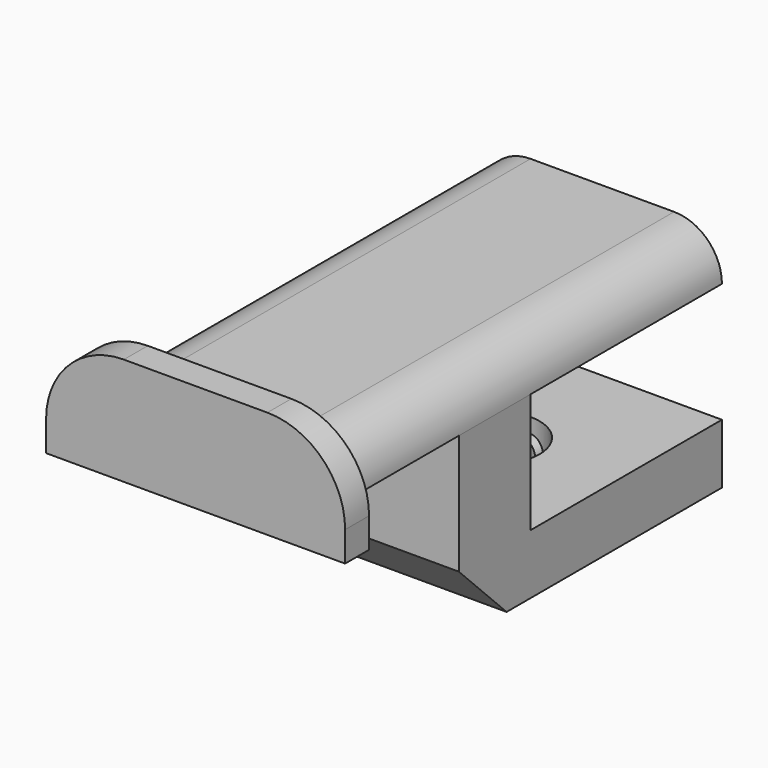
from build123d import *

# Parameters (mm, degrees)
F0_W      = 40
F0_H      = 80
F1_DEPTH  = 8
F2_W      = 40
F2_H      = 15
F3_DEPTH  = 30
F4_W      = 40
F4_H      = 10
F5_DEPTH  = 40
F6_R      = 7.99999
F7_SIZE2  = 10
F7_SIZE   = 10
F9_DEPTH  = 5
F10_W     = 48
F10_H     = 5
F10_W_2   = 1
F11_DEPTH = 5
F12_R     = 7.5
F12_R_2   = 6
F13_DEPTH = 11
F14_R     = 2.5
F15_DEPTH = 32
F16_DEPTH = 25


# Not quite as in the source:
# - a fillet or chamfer is up to 0.001 mm smaller than in the source, because OpenCascade refuses the exact size


with BuildPart() as f1:
    # F0 (on Top) → F1 (new body)
    with BuildSketch(Plane.XY):
        with Locations((-20, 2.0996452868)):
            Rectangle(F0_W, F0_H)
    extrude(amount=F1_DEPTH)

    # F2 (on face) → F3 (join)
    with BuildSketch(Plane(origin=(0, 0, 0), x_dir=(1, 0, 0), z_dir=(0, 0, -1))):
        with Locations((-20, 5.4003547132)):
            Rectangle(F2_W, F2_H)
    extrude(amount=F3_DEPTH)

    # F4 (on face) → F5 (join)
    with BuildSketch(Plane(origin=(0, 2.0996452868, 0), x_dir=(-1, 0, 0), z_dir=(0, 1, 0))):
        with Locations((20, -25)):
            Rectangle(F4_W, F4_H)
    extrude(amount=F5_DEPTH)

    # F6 (radius 8 in the source; OpenCascade refuses exactly that, so slightly less here)
    f6_edges = [f1.edges().sort_by_distance(p)[0] for p in [
        (0, 2.099645, 8),
        (-40, 2.099645, 8),
    ]]
    fillet(f6_edges, radius=F6_R)

    # F7
    f7_edges = [f1.edges().sort_by_distance(p)[0] for p in [
        (-20, -12.900355, -30),
    ]]
    chamfer(f7_edges, length=F7_SIZE, length2=F7_SIZE2)

    # F8 (on face) → F9 (join)
    with BuildSketch(Plane.XZ.offset(37.9003547132)):
        with BuildLine():
            Line((-44, -5), (4, -5))
            ThreePointArc((4, -5), (2.8166538264, 7.2111025509), (-8, 13))
            Line((-8, 13), (-32, 13))
            ThreePointArc((-32, 13), (-42.8166538264, 7.2111025509), (-44, -5))
        make_face()
    extrude(amount=F9_DEPTH)

    # F10 (on face) → F11 (join)
    with BuildSketch(Plane(origin=(0, 0, -5), x_dir=(1, 0, 0), z_dir=(0, 0, -1))):
        with Locations((-20, 40.4003547132)):
            Rectangle(F10_W, F10_H)
        with Locations((-44.5, 40.4003547132)):
            Rectangle(F10_W_2, F10_H)
        with Locations((4.5, 40.4003547132)):
            Rectangle(F10_W_2, F10_H)
    extrude(amount=-F11_DEPTH)

    # F12 (on face) → F13 (cut)
    with BuildSketch(Plane(origin=(0, 0, -30), x_dir=(1, 0, 0), z_dir=(0, 0, -1))):
        with Locations((-20, -19.5996452868)):
            Circle(F12_R)
        with Locations((-20, -19.5996452868)):
            Circle(F12_R_2, mode=Mode.SUBTRACT)
        with Locations((-20, -19.5996452868)):
            Circle(F12_R_2)
    extrude(amount=-F13_DEPTH, mode=Mode.SUBTRACT)

    # F14 (on face) → F15 (join)
    with BuildSketch(Plane(origin=(0, 42.0996452868, 0), x_dir=(-1, 0, 0), z_dir=(0, 1, 0))):
        with Locations((20, -25)):
            Circle(F14_R)
    extrude(amount=-F15_DEPTH)

    # F12 (on face) → F16 (cut)
    with BuildSketch(Plane(origin=(0, 0, -30), x_dir=(1, 0, 0), z_dir=(0, 0, -1))):
        with Locations((-20, -19.5996452868)):
            Circle(F12_R_2)
    extrude(amount=-F16_DEPTH, mode=Mode.SUBTRACT)


solid = f1.part
